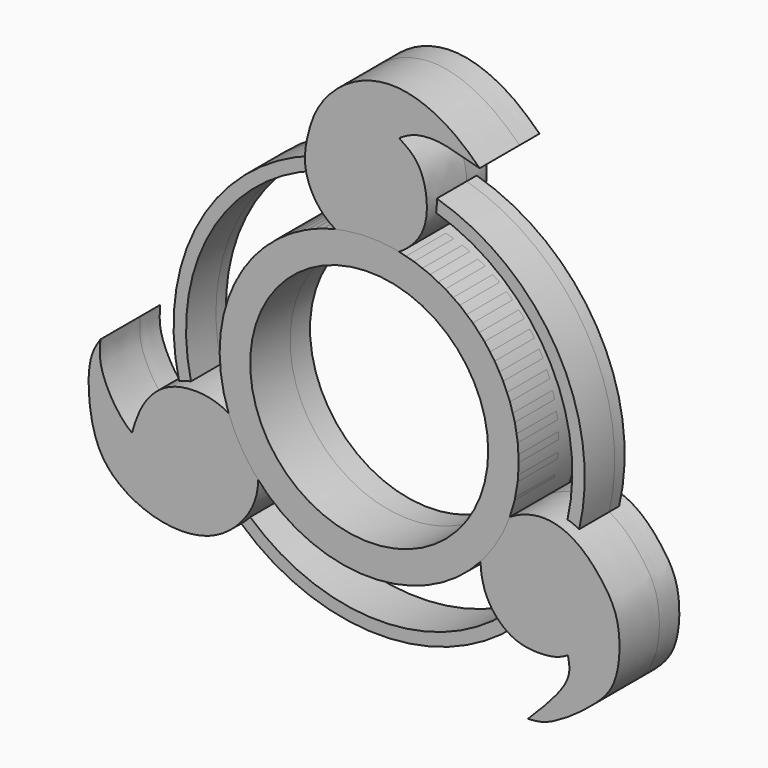
from build123d import *

# Parameters (mm, degrees)
F1_R        = 20.955
F1_R_2      = 19.685
F2_DEPTH    = 3.81
F0_R        = 15.24
F0_R_2      = 12.1285
F3_DEPTH    = 5.08
F5_DEPTH    = 5.08
F3_FACE_R   = 15.24
F3_FACE_R_2 = 12.1285
F6_DEPTH    = 7.62
F7_DEPTH    = 5.08


with BuildPart() as f2:
    # F1 (on Front) → F2 (new body)
    with BuildSketch(Plane.XZ):
        Circle(F1_R)
        Circle(F1_R_2, mode=Mode.SUBTRACT)
    extrude(amount=F2_DEPTH)

    # F4 (on Front) → F5 (join)
    with BuildSketch(Plane.XZ):
        with BuildLine():
            add(Edge.make_bspline(
                [(20.2570147812, -15.6700648367), (19.8961694208, -15.8805236851), (19.0041175108, -16.4008025587), (15.8720621479, -16.559826062), (13.5312359314, -15.4147247099), (11.7272072425, -13.1399714713), (11.2166446038, -10.2137107801), (11.4999702986, -7.6218597128), (14.3865819004, -4.722269119), (18.1587165263, -3.7797428799), (21.4460389306, -5.1940456945), (23.8429017776, -7.8661286141), (25.6734991364, -10.8199724294), (25.5377481708, -16.3390016258), (23.2461494272, -19.2023701616), (18.452391334, -22.5753039632), (16.8043370097, -22.6711036419), (16.1752011627, -22.7076746523)],
                knots=[0, 0, 0, 0, 0.0436885344, 0.1080031639, 0.1676295863, 0.2294719046, 0.2924472264, 0.3509340914, 0.4237263668, 0.4953038566, 0.5634406065, 0.6326971489, 0.7017391482, 0.7852820259, 0.857371763, 0.94555244, 1, 1, 1, 1], degree=3))
            add(Edge.make_bspline(
                [(20.2570147812, -15.6700648367), (20.3829041644, -16.3084867464), (20.6845521254, -17.838231848), (17.9411549431, -20.9485961903), (16.7201363375, -22.1648610522), (16.1752011627, -22.7076746523)],
                knots=[0, 0, 0, 0, 0.2839743748, 0.6804409471, 1, 1, 1, 1], degree=3))
        make_face()
        with BuildLine():
            add(Edge.make_bspline(
                [(3.0488960911, 25.1434091479), (3.7182536947, 24.6990821502), (5.1726496809, 23.7336379712), (6.1241493354, 20.3115195563), (5.5613721245, 16.69225876), (2.0341131265, 13.9757621792), (-1.5557545968, 13.7470005644), (-5.0342055625, 15.5452774991), (-6.8469141166, 19.2212913575), (-6.3055975072, 22.4630575555), (-5.3424365083, 25.5025980603), (-2.1010733373, 28.9284126178), (3.0910934799, 30.2162430426), (8.3134253187, 27.9097705394), (10.3284132794, 25.9855691321), (11.2594394013, 25.0964909792)],
                knots=[0, 0, 0, 0, 0.0616302497, 0.1339116599, 0.2079808628, 0.2881086137, 0.361437359, 0.4374817635, 0.5149936036, 0.5852235295, 0.6550849429, 0.7387987633, 0.8281216337, 0.9205835211, 1, 1, 1, 1], degree=3))
            add(Edge.make_bspline(
                [(11.2594394013, 25.0964909792), (10.5646308324, 25.2820628254), (9.1428071033, 25.6618083644), (6.8452879901, 26.2699311214), (4.5200290319, 26.0390563832), (3.5142351531, 25.4267143698), (3.0488960911, 25.1434091479)],
                knots=[0, 0, 0, 0, 0.2537571195, 0.5192766902, 0.7775892867, 1, 1, 1, 1], degree=3))
        make_face()
        with BuildLine():
            add(Edge.make_bspline(
                [(-27.3906067014, -2.8257619124), (-27.790953611, -3.4332696992), (-28.8075634718, -4.9759278086), (-28.5233011705, -10.9489031163), (-26.5289063724, -14.867132619), (-21.7070990271, -17.5170081944), (-15.8617714826, -17.4320795969), (-11.8371266697, -13.6636122638), (-10.8215735606, -9.3413615315), (-13.4799514164, -5.1719896976), (-17.2969878336, -4.0269277312), (-21.0629413694, -4.6828120412), (-23.3644095401, -7.4279222295), (-23.9139992286, -9.2808253639), (-24.1766812534, -10.1669620555)],
                knots=[0, 0, 0, 0, 0.0636228496, 0.1615589249, 0.2469563528, 0.340002317, 0.4365777254, 0.5291519495, 0.6119248419, 0.6984248894, 0.7782692107, 0.8560101465, 0.9311136098, 0.9999516489, 0.9999516489, 0.9999516489, 0.9999516489], degree=3))
            add(Edge.make_bspline(
                [(-24.1766812534, -10.1669620555), (-24.3509354034, -10.0365492919), (-24.9137715031, -9.5865420103), (-26.1827320151, -8.0804292282), (-27.5785954401, -5.1680066439), (-27.4497008963, -3.5620457329), (-27.3906067014, -2.8257619124)],
                knots=[0.058079573, 0.058079573, 0.058079573, 0.058079573, 0.175325606, 0.4277692031, 0.7376497308, 1, 1, 1, 1], degree=3))
        make_face()
    extrude(amount=F5_DEPTH)

    # F5_face (on face) + F3_face (on face) → F6 (join)
    with BuildSketch(Plane(origin=(0.3501446765, -5.08, 21.9228061941), x_dir=(1, 0, 0), z_dir=(0, -1, 0))):
        with BuildLine():
            add(Edge.make_bspline(
                [(2.6987514145, 3.2206029537), (3.3681090182, 2.776275956), (4.8225050044, 1.8108317771), (5.7740046589, -1.6112866378), (5.2112274479, -5.2305474341), (1.68396845, -7.9470440149), (-1.9058992733, -8.1758056297), (-5.3843502391, -6.3775286951), (-7.1970587932, -2.7015148366), (-6.6557421837, 0.5402513614), (-5.6925811848, 3.5797918662), (-2.4512180138, 7.0056064236), (2.7409488034, 8.2934368484), (7.9632806422, 5.9869643453), (9.9782686029, 4.062762938), (10.9092947248, 3.1736847851)],
                knots=[0, 0, 0, 0, 0.0616302497, 0.1339116599, 0.2079808628, 0.2881086137, 0.361437359, 0.4374817635, 0.5149936036, 0.5852235295, 0.6550849429, 0.7387987633, 0.8281216337, 0.9205835211, 1, 1, 1, 1], degree=3))
            add(Edge.make_bspline(
                [(10.9092947248, 3.1736847851), (10.2144861559, 3.3592566313), (8.7926624268, 3.7390021703), (6.4951433136, 4.3471249273), (4.1698843554, 4.1162501891), (3.1640904766, 3.5039081757), (2.6987514145, 3.2206029537)],
                knots=[0, 0, 0, 0, 0.2537571195, 0.5192766902, 0.7775892867, 1, 1, 1, 1], degree=3))
        make_face()
        with BuildLine():
            add(Edge.make_bspline(
                [(-24.5268259299, -32.0897682496), (-24.7010800799, -31.959355486), (-25.2639161796, -31.5093482044), (-26.5328766916, -30.0032354224), (-27.9287401166, -27.090812838), (-27.7998455728, -25.484851927), (-27.7407513779, -24.7485681065)],
                knots=[0.058079573, 0.058079573, 0.058079573, 0.058079573, 0.175325606, 0.4277692031, 0.7376497308, 1, 1, 1, 1], degree=3))
            add(Edge.make_bspline(
                [(-27.7407513779, -24.7485681065), (-28.1410982875, -25.3560758933), (-29.1577081484, -26.8987340027), (-28.873445847, -32.8717093104), (-26.8790510489, -36.7899388131), (-22.0572437036, -39.4398143885), (-16.2119161591, -39.354885791), (-12.1872713462, -35.586418458), (-11.1717182371, -31.2641677256), (-13.8300960929, -27.0947958917), (-17.6471325101, -25.9497339253), (-21.4130860459, -26.6056182354), (-23.7145542167, -29.3507284237), (-24.2641439051, -31.203631558), (-24.5268259299, -32.0897682496)],
                knots=[0, 0, 0, 0, 0.0636228496, 0.1615589249, 0.2469563528, 0.340002317, 0.4365777254, 0.5291519495, 0.6119248419, 0.6984248894, 0.7782692107, 0.8560101465, 0.9311136098, 0.9999516489, 0.9999516489, 0.9999516489, 0.9999516489], degree=3))
        make_face()
        with BuildLine():
            add(Edge.make_bspline(
                [(19.9068701047, -37.5928710309), (19.5460247443, -37.8033298792), (18.6539728343, -38.3236087528), (15.5219174714, -38.4826322561), (13.1810912549, -37.337530904), (11.377062566, -35.0627776654), (10.8664999273, -32.1365169742), (11.1498256221, -29.544665907), (14.0364372239, -26.6450753131), (17.8085718498, -25.702549074), (21.0958942541, -27.1168518886), (23.4927571011, -29.7889348082), (25.3233544599, -32.7427786235), (25.1876034943, -38.2618078199), (22.8960047507, -41.1251763557), (18.1022466575, -44.4981101573), (16.4541923332, -44.593909836), (15.8250564862, -44.6304808465)],
                knots=[0, 0, 0, 0, 0.0436885344, 0.1080031639, 0.1676295863, 0.2294719046, 0.2924472264, 0.3509340914, 0.4237263668, 0.4953038566, 0.5634406065, 0.6326971489, 0.7017391482, 0.7852820259, 0.857371763, 0.94555244, 1, 1, 1, 1], degree=3))
            add(Edge.make_bspline(
                [(19.9068701047, -37.5928710309), (20.0327594879, -38.2312929405), (20.3344074489, -39.7610380421), (17.5910102666, -42.8714023844), (16.369991661, -44.0876672463), (15.8250564862, -44.6304808465)],
                knots=[0, 0, 0, 0, 0.2839743748, 0.6804409471, 1, 1, 1, 1], degree=3))
        make_face()
    with BuildSketch(Plane.XZ.offset(5.08)):
        Circle(F3_FACE_R)
        Circle(F3_FACE_R_2, mode=Mode.SUBTRACT)
    extrude(amount=-F6_DEPTH)

    # F7 (add): faces of the model
    f7_faces = [f2.faces().sort_by_distance(p)[0] for p in [
        (-0.0072632879, -3.81, -20.666980446),
        (19.9126140007, -3.81, -4.300047256),
        (-6.7569038247, -3.81, 19.2204268278),
    ]]
    extrude(f7_faces, amount=-F7_DEPTH)


with BuildPart() as f3:
    # F0 (on Front) → F3 (new body)
    with BuildSketch(Plane.XZ):
        Circle(F0_R)
        Circle(F0_R_2, mode=Mode.SUBTRACT)
    extrude(amount=F3_DEPTH)


solid = Compound([f2.part, f3.part])
